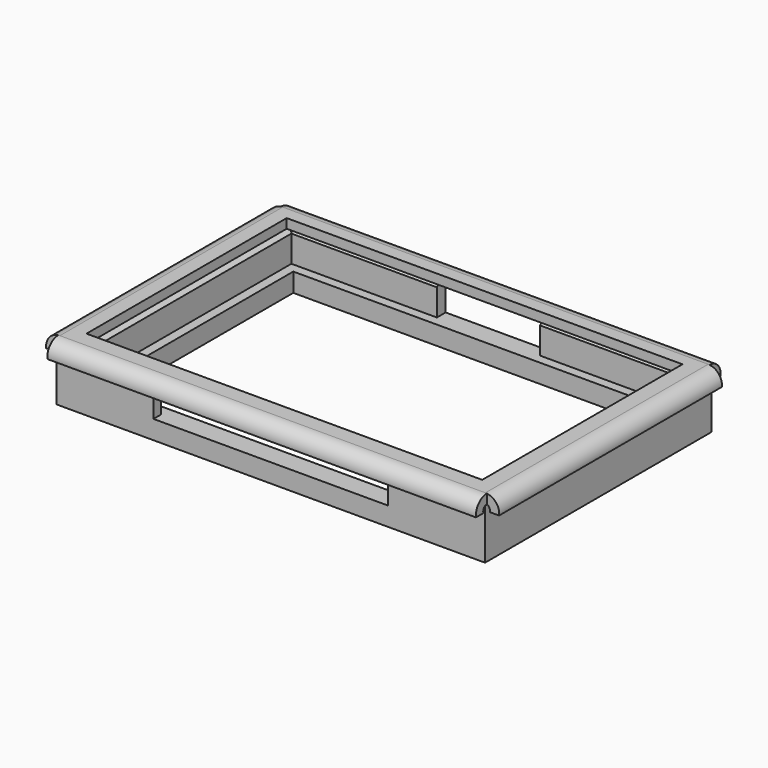
from build123d import *

# Parameters (mm, degrees)
F0_W      = 137
F0_H      = 90.5
F0_W_2    = 120.5
F0_H_2    = 77.5
F1_DEPTH  = 16
F3_W      = 33
F3_H      = 39.131847919
F3_H_2    = 13
F3_W_2    = 75
F3_H_3    = 13.5
F3_H_4    = 6.5
F4_DEPTH  = 10
F5_SIZE   = 1.5
F6_R      = 1.55
F7_DEPTH  = 3
F8_DEPTH  = 3
F9_W      = 136
F9_H      = 3
F10_DEPTH = 44.5
F12_DEPTH = 68.5
F13_W     = 126.5
F13_H     = 80
F14_DEPTH = 10
F15_DEPTH = 3


# Not quite as in the source:
# - a feature names something its author has since deleted; it is built from what else it names


with BuildPart() as f1:
    # F0 (on Top) → F1 (new body)
    with BuildSketch(Plane.XY):
        Rectangle(F0_W, F0_H)
        with Locations((0.25, 0)):
            Rectangle(F0_W_2, F0_H_2, mode=Mode.SUBTRACT)
    extrude(amount=F1_DEPTH)

    # F3 (on 3pt) → F4 (cut)
    with BuildSketch(Plane.XY.offset(16)):
        with Locations((0, 61.3159239595)):
            Rectangle(F3_W, F3_H)
        with Locations((0, 35.25)):
            Rectangle(F3_W, F3_H_2)
        Polygon((-16.5, 28.75), (-16.5, 41.75), (-63, 41.75), (-63, -37.25), (-58, -42.25), (-37.5, -42.25), (-37.5, -28.75), (37.5, -28.75), (37.5, -42.25), (58.5, -42.25), (63.5, -37.25), (63.5, 36.75), (58.5, 41.75), (16.5, 41.75), (16.5, 28.75), align=None)
        with Locations((0, -35.5)):
            Rectangle(F3_W_2, F3_H_3)
        with Locations((0, -45.5)):
            Rectangle(F3_W_2, F3_H_4)
    extrude(amount=-F4_DEPTH, mode=Mode.SUBTRACT)

    # F5
    f5_edges = [f1.edges().sort_by_distance(p)[0] for p in [
        (-63, 2.25, 16),
        (-39.75, 41.75, 16),
        (61, 39.25, 16),
        (63.5, -0.25, 16),
        (61, -39.75, 16),
        (-60.5, -39.75, 16),
        (-47.75, -42.25, 16),
        (48, -42.25, 16),
        (37.5, 41.75, 16),
    ]]
    chamfer(f5_edges, length=F5_SIZE)

    # F6 (on face) → F7 (cut)
    with BuildSketch(Plane.XY.offset(16)):
        with Locations((-66.15, 42.75)):
            Circle(F6_R)
        with Locations((-65.5, -42.25)):
            Circle(F6_R)
        with Locations((66, -42.25)):
            Circle(F6_R)
        with Locations((64.7276754423, 42.15)):
            Circle(F6_R)
    extrude(amount=-F7_DEPTH, mode=Mode.SUBTRACT)


with BuildPart() as f8:
    # F6 (on face) → F8 (new body)
    with BuildSketch(Plane.XY.offset(16)):
        with Locations((-66.15, 42.75)):
            Circle(F6_R)
    extrude(amount=-F8_DEPTH)


with BuildPart() as f8b:
    # F6 (on face) → F8, piece 2 (new body)
    with BuildSketch(Plane.XY.offset(16)):
        with Locations((-65.5, -42.25)):
            Circle(F6_R)
    extrude(amount=-F8_DEPTH)


with BuildPart() as f8c:
    # F6 (on face) → F8, piece 3 (new body)
    with BuildSketch(Plane.XY.offset(16)):
        with Locations((66, -42.25)):
            Circle(F6_R)
    extrude(amount=-F8_DEPTH)


with BuildPart() as f8d:
    # F6 (on face) → F8, piece 4 (new body)
    with BuildSketch(Plane.XY.offset(16)):
        with Locations((64.7276754423, 42.15)):
            Circle(F6_R)
    extrude(amount=-F8_DEPTH)


with BuildPart() as f10:
    # F9 (on Front) → F10 (new body, symmetric)
    with BuildSketch(Plane.XZ):
        with Locations((0, 17.7)):
            Rectangle(F9_W, F9_H)
        with BuildLine():
            Line((-68, 16.2), (-68, 19.2))
            ThreePointArc((-68, 19.2), (-71.3106094408, 17.7056160116), (-72.3797211221, 14.2342591319))
            Line((-72.3797211221, 14.2342591319), (-69.3797211221, 14.2342591319))
            ThreePointArc((-69.3797211221, 14.2342591319), (-69.2008088457, 15.575755747), (-68, 16.2))
        make_face()
        with BuildLine():
            ThreePointArc((72.3797211221, 14.2342591319), (71.3106094408, 17.7056160116), (68, 19.2))
            Line((68, 19.2), (68, 16.2))
            ThreePointArc((68, 16.2), (69.2008088457, 15.575755747), (69.3797211221, 14.2342591319))
            Line((69.3797211221, 14.2342591319), (72.3797211221, 14.2342591319))
        make_face()
    extrude(amount=F10_DEPTH, both=True)

    # F11 (on Right) → F12 (join, symmetric)
    with BuildSketch(Plane.YZ):
        with BuildLine():
            ThreePointArc((48.8797211221, 14.2342591319), (47.8106094408, 17.7056160116), (44.5, 19.2))
            Line((44.5, 19.2), (44.5, 16.2))
            ThreePointArc((44.5, 16.2), (45.7165581841, 15.5868099481), (45.8797211221, 14.2342591319))
            Line((45.8797211221, 14.2342591319), (48.8797211221, 14.2342591319))
        make_face()
        with BuildLine():
            ThreePointArc((-44.5, 19.2), (-47.8106094408, 17.7056160116), (-48.8797211221, 14.2342591319))
            Line((-48.8797211221, 14.2342591319), (-45.8797211221, 14.2342591319))
            ThreePointArc((-45.8797211221, 14.2342591319), (-45.7165581841, 15.5868099481), (-44.5, 16.2))
            Line((-44.5, 16.2), (-44.5, 19.2))
        make_face()
    extrude(amount=F12_DEPTH, both=True)

    # F13 (on face) → F14 (cut)
    with BuildSketch(Plane.XY.offset(19.2)):
        with Locations((-0.25, 0.5)):
            Rectangle(F13_W, F13_H)
    extrude(amount=-F14_DEPTH, mode=Mode.SUBTRACT)

    # F6 (on face) → F15 (cut)
    with BuildSketch(Plane.XY.offset(16)):
        with Locations((-66.15, 42.75)):
            Circle(F6_R)
        with Locations((-65.5, -42.25)):
            Circle(F6_R)
        with Locations((66, -42.25)):
            Circle(F6_R)
        with Locations((64.7276754423, 42.15)):
            Circle(F6_R)
    extrude(amount=F15_DEPTH, mode=Mode.SUBTRACT)


solid = Compound([f1.part, f8.part, f8b.part, f8c.part, f8d.part, f10.part])
